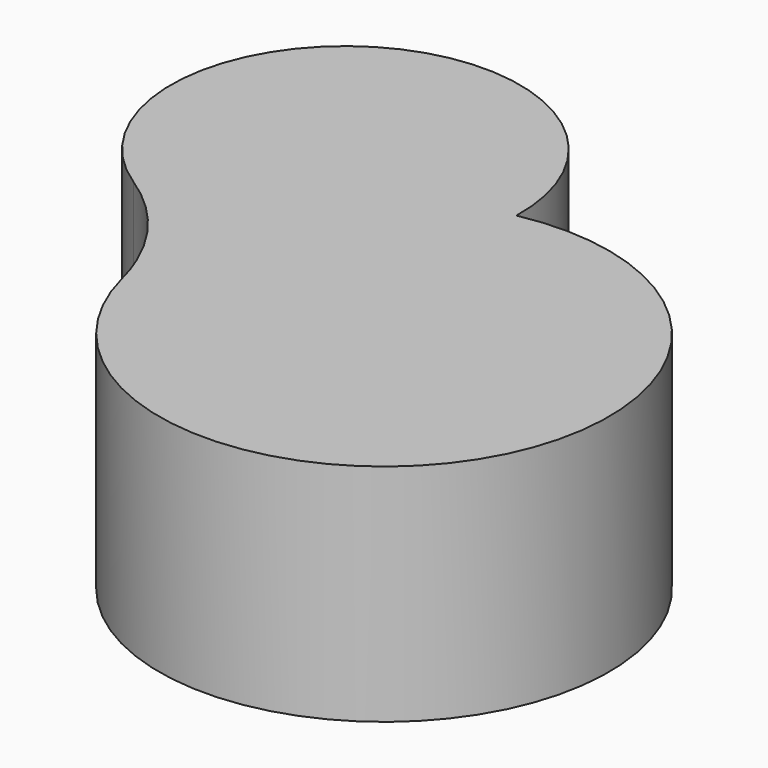
from build123d import *

# Parameters (mm, degrees)
F1_DEPTH = 20
F2_R     = 20


# Not quite as in the source:
# - the program builds the solid bodies; features that only make, move or delete a surface that nothing else refers to are left out


with BuildPart() as f1:
    # F0 (on Top) → F1 (new body)
    with BuildSketch(Plane.XY):
        with BuildLine():
            ThreePointArc((-3.9175447913, 19.6125684909), (-30.2449014117, 31.1090570268), (-19.494455089, 4.4683577278))
            ThreePointArc((-19.494455089, 4.4683577278), (13.9415642776, -14.3399018648), (-3.9175447913, 19.6125684909))
        make_face()
    extrude(amount=F1_DEPTH)

    # F2
    f2_edges = [f1.edges().sort_by_distance(p)[0] for p in [
        (-19.494455, 4.468358, 10),
    ]]
    fillet(f2_edges, radius=F2_R)


solid = f1.part
